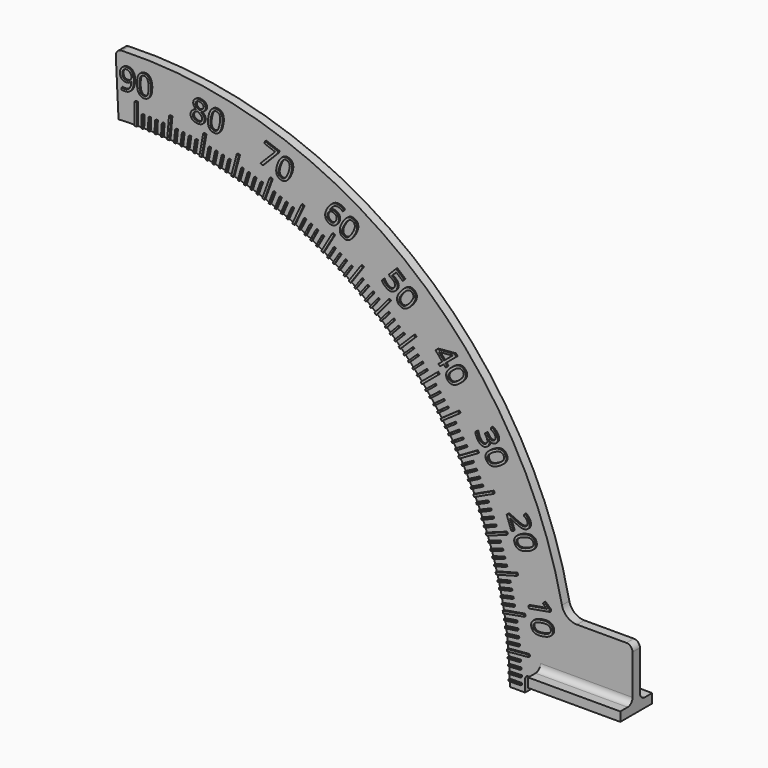
from build123d import *

# Parameters (mm, degrees)
F2_DEPTH     = 1.5
F0_TEXT_SIZE = 9.7222222222
F3_DEPTH     = 2
F4_W         = 30
F4_H         = 3
F5_DEPTH     = 6.5
F6_R         = 2


# Not quite as in the source:
# - Text() gives the source's letters only with a copy of the font that has no kerning and outlines rounded to 1/6400 em; it was checked with that copy


with BuildPart() as f2:
    # F1 (on Front) → F2 (new body, symmetric)
    with BuildSketch(Plane.XZ):
        with BuildLine():
            ThreePointArc((0, 121.5), (85.9134739142, 85.9134739142), (121.5, 0))
            Line((121.5, 0), (126.5, 0))
            Line((126.5, 0), (126.5, 4))
            ThreePointArc((126.5, 4), (126.7928932188, 4.7071067812), (127.5, 5))
            Line((127.5, 5), (161.5, 5))
            Line((161.5, 5), (161.5, 23))
            ThreePointArc((161.5, 23), (160.9142135624, 24.4142135624), (159.5, 25))
            Line((159.5, 25), (143.3954322843, 25))
            ThreePointArc((143.3954322843, 25), (140.2426124294, 26.1193135965), (138.5013902268, 28.976109215))
            ThreePointArc((138.5013902268, 28.976109215), (87.2865254437, 111.3701597196), (-4.9586057544, 141.413090727))
            ThreePointArc((-4.9586057544, 141.413090727), (-6.3611618138, 140.7675835059), (-6.8860808014, 139.315583806))
            Line((-6.8860808014, 139.315583806), (-5.9981707317, 121.3518518519))
            ThreePointArc((-5.9981707317, 121.3518518519), (-3, 121.4629573162), (0, 121.5))
        make_face()
    extrude(amount=F2_DEPTH, both=True)

    # F0 (on Front) → F3 (join)
    with BuildSketch(Plane.XZ):
        with BuildLine():
            ThreePointArc((0.25, 121.4997427981), (0.3000000254, 121.499629629), (0.35, 121.4994958837))
            Line((0.35, 121.4994958837), (0.35, 128.5))
            Line((0.35, 128.5), (-0.35, 128.5))
            Line((-0.35, 128.5), (-0.35, 121.4994958837))
            ThreePointArc((-0.35, 121.4994958837), (-0.3000000254, 121.499629629), (-0.25, 121.4997427981))
            Line((-0.25, 121.4997427981), (-0.25, 125.5))
            Line((-0.25, 125.5), (0.25, 125.5))
            Line((0.25, 125.5), (0.25, 121.4997427981))
        make_face()
        with BuildLine():
            ThreePointArc((1.8705009695, 121.4856009004), (2.1204673821, 121.4814949615), (2.3704248171, 121.4768746971))
            Line((2.3704248171, 121.4768746971), (2.4402389317, 125.4765226405))
            Line((2.4402389317, 125.4765226405), (1.9403150841, 125.4852488437))
            Line((1.9403150841, 125.4852488437), (1.8705009695, 121.4856009004))
        make_face()
        with BuildLine():
            ThreePointArc((3.9904321664, 121.4344533118), (4.2402888494, 121.4259854828), (4.4901275799, 121.4170035634))
            Line((4.4901275799, 121.4170035634), (4.6297345429, 125.4148239167))
            Line((4.6297345429, 125.4148239167), (4.1300391294, 125.4322736651))
            Line((4.1300391294, 125.4322736651), (3.9904321664, 121.4344533118))
        make_face()
        with BuildLine():
            ThreePointArc((6.1091478389, 121.3463156123), (6.3588186835, 121.3334884727), (6.6084626063, 121.3201476342))
            Line((6.6084626063, 121.3201476342), (6.8178198922, 125.3149226226))
            Line((6.8178198922, 125.3149226226), (6.3185051248, 125.3410906008))
            Line((6.3185051248, 125.3410906008), (6.1091478389, 121.3463156123))
        make_face()
        with BuildLine():
            ThreePointArc((8.2260026058, 121.2212146496), (8.4754115599, 121.2040321066), (8.724784631, 121.1863364127))
            Line((8.724784631, 121.1863364127), (9.0038284675, 125.1768491892))
            Line((9.0038284675, 125.1768491892), (8.5050464423, 125.211727426))
            Line((8.5050464423, 125.211727426), (8.2260026058, 121.2212146496))
        make_face()
        with BuildLine():
            ThreePointArc((10.2407106629, 121.0676581302), (10.5894227438, 121.0376558181), (10.9380469515, 121.0066491102))
            Line((10.9380469515, 121.0066491102), (11.5481810874, 127.9805141948))
            Line((11.5481810874, 127.9805141948), (10.8508447987, 128.0415232148))
            Line((10.8508447987, 128.0415232148), (10.2407106629, 121.0676581302))
        make_face()
        with BuildLine():
            ThreePointArc((12.4515509283, 120.8602866101), (12.700208287, 120.8344102872), (12.9488118759, 120.8080223785))
            Line((12.9488118759, 120.8080223785), (13.3669526139, 124.7863657529))
            Line((13.3669526139, 124.7863657529), (12.8696916662, 124.8386299845))
            Line((12.8696916662, 124.8386299845), (12.4515509283, 120.8602866101))
        make_face()
        with BuildLine():
            ThreePointArc((14.5589573408, 120.6245694755), (14.8071252237, 120.5943574244), (15.0552304166, 120.5636348038))
            Line((15.0552304166, 120.5636348038), (15.5427391353, 124.5340746951))
            Line((15.5427391353, 124.5340746951), (15.0464660594, 124.5950093668))
            Line((15.0464660594, 124.5950093668), (14.5589573408, 120.6245694755))
        make_face()
        with BuildLine():
            ThreePointArc((16.6619289539, 120.3521089285), (16.9095317666, 120.3175703521), (17.1570629882, 120.282522378))
            Line((17.1570629882, 120.282522378), (17.7137911877, 124.2438493518))
            Line((17.7137911877, 124.2438493518), (17.2186571533, 124.3134359023))
            Line((17.2186571533, 124.3134359023), (16.6619289539, 120.3521089285))
        make_face()
        with BuildLine():
            ThreePointArc((18.759825182, 120.0429879632), (19.0067875024, 120.0041333823), (19.2536693523, 119.9647707307))
            Line((19.2536693523, 119.9647707307), (19.8794474477, 123.9157781284))
            Line((19.8794474477, 123.9157781284), (19.3856032774, 123.9939953609))
            Line((19.3856032774, 123.9939953609), (18.759825182, 120.0429879632))
        make_face()
        with BuildLine():
            ThreePointArc((20.7534833341, 119.7144223956), (21.0982535865, 119.654141991), (21.4428487612, 119.5928686712))
            Line((21.4428487612, 119.5928686712), (22.6584735438, 126.4870193999))
            Line((22.6584735438, 126.4870193999), (21.9691081166, 126.6085731243))
            Line((21.9691081166, 126.6085731243), (20.7534833341, 119.7144223956))
        make_face()
        with BuildLine():
            ThreePointArc((22.9378370659, 119.3151525613), (23.1832929383, 119.2677027889), (23.4286506577, 119.2197480637))
            Line((23.4286506577, 119.2197480637), (24.1919357156, 123.1465092738))
            Line((24.1919357156, 123.1465092738), (23.7011221239, 123.2419137715))
            Line((23.7011221239, 123.2419137715), (22.9378370659, 119.3151525613))
        make_face()
        with BuildLine():
            ThreePointArc((25.0166800589, 118.8966598304), (25.2612704344, 118.8449334892), (25.5057538593, 118.792703985))
            Line((25.5057538593, 118.792703985), (26.3374540978, 122.7055459694))
            Line((26.3374540978, 122.7055459694), (25.8483802974, 122.8095018148))
            Line((25.8483802974, 122.8095018148), (25.0166800589, 118.8966598304))
        make_face()
        with BuildLine():
            ThreePointArc((27.0879027287, 118.4419500251), (27.3315531028, 118.3859628714), (27.5750877611, 118.329474498))
            Line((27.5750877611, 118.329474498), (28.4749498364, 122.227205367))
            Line((28.4749498364, 122.227205367), (27.987764804, 122.3396808941))
            Line((27.987764804, 122.3396808941), (27.0879027287, 118.4419500251))
        make_face()
        with BuildLine():
            ThreePointArc((29.150874161, 117.9511616545), (29.3935103154, 117.8909307425), (29.6360220242, 117.8302007067))
            Line((29.6360220242, 117.8302007067), (30.6037718293, 121.7116331737))
            Line((30.6037718293, 121.7116331737), (30.1186239662, 121.8325941215))
            Line((30.1186239662, 121.8325941215), (29.150874161, 117.9511616545))
        make_face()
        with BuildLine():
            ThreePointArc((31.1083094659, 117.450087621), (31.44651398, 117.3599878941), (31.7844575443, 117.2689142894))
            Line((31.7844575443, 117.2689142894), (33.5963213349, 124.0308820124))
            Line((33.5963213349, 124.0308820124), (32.9201732565, 124.2120553439))
            Line((32.9201732565, 124.2120553439), (31.1083094659, 117.450087621))
        make_face()
        with BuildLine():
            ThreePointArc((33.2495524133, 116.8619581571), (33.4899387318, 116.7932960565), (33.7301832613, 116.7241394792))
            Line((33.7301832613, 116.7241394792), (34.832803579, 120.5694335013))
            Line((34.832803579, 120.5694335013), (34.352172731, 120.7072521792))
            Line((34.352172731, 120.7072521792), (33.2495524133, 116.8619581571))
        make_face()
        with BuildLine():
            ThreePointArc((35.2840107363, 116.2638748123), (35.5231621238, 116.1910278495), (35.7621631142, 116.1176889599))
            Line((35.7621631142, 116.1176889599), (36.9317251317, 119.9431539472))
            Line((36.9317251317, 119.9431539472), (36.4535727537, 120.0893397995))
            Line((36.4535727537, 120.0893397995), (35.2840107363, 116.2638748123))
        make_face()
        with BuildLine():
            ThreePointArc((37.3077212077, 115.6303763649), (37.5455648166, 115.5533667299), (37.7832494659, 115.4758678677))
            Line((37.7832494659, 115.4758678677), (39.0193969231, 119.2803385464))
            Line((39.0193969231, 119.2803385464), (38.543868665, 119.4348470436))
            Line((38.543868665, 119.4348470436), (37.3077212077, 115.6303763649))
        make_face()
        with BuildLine():
            ThreePointArc((39.3200673859, 114.9616557847), (39.5565307665, 114.8805069353), (39.7928266737, 114.7988717075))
            Line((39.7928266737, 114.7988717075), (41.0951830283, 118.5811891991))
            Line((41.0951830283, 118.5811891991), (40.6224237405, 118.7439732763))
            Line((40.6224237405, 118.7439732763), (39.3200673859, 114.9616557847))
        make_face()
        with BuildLine():
            ThreePointArc((41.2263825789, 114.2918867613), (41.5554474141, 114.1726534255), (41.8841674134, 114.052472661))
            Line((41.8841674134, 114.052472661), (44.2784808346, 120.6307947208))
            Line((44.2784808346, 120.6307947208), (43.620696, 120.8702088212))
            Line((43.620696, 120.8702088212), (41.2263825789, 114.2918867613))
        make_face()
        with BuildLine():
            ThreePointArc((43.3082185902, 113.5193736881), (43.5417058698, 113.4300218194), (43.7750088035, 113.3401897133))
            Line((43.7750088035, 113.3401897133), (45.2085727746, 117.074751538))
            Line((45.2085727746, 117.074751538), (44.7417825613, 117.2539355128))
            Line((44.7417825613, 117.2539355128), (43.3082185902, 113.5193736881))
        make_face()
        with BuildLine():
            ThreePointArc((45.2828087869, 112.7462515048), (45.5147011, 112.6528383299), (45.7464007141, 112.558948208))
            Line((45.7464007141, 112.558948208), (47.2449234373, 116.2679220998))
            Line((47.2449234373, 116.2679220998), (46.7813315101, 116.4552253965))
            Line((46.7813315101, 116.4552253965), (45.2828087869, 112.7462515048))
        make_face()
        with BuildLine():
            ThreePointArc((47.2436054013, 111.938785721), (47.4738321114, 111.8413396945), (47.703857828, 111.7434201567))
            Line((47.703857828, 111.7434201567), (49.2668828388, 115.4256763262))
            Line((49.2668828388, 115.4256763262), (48.806630412, 115.6210418904))
            Line((48.806630412, 115.6210418904), (47.2436054013, 111.938785721))
        make_face()
        with BuildLine():
            ThreePointArc((49.1900111559, 111.0972222987), (49.4185021337, 110.9957731036), (49.6467838847, 110.8938539772))
            Line((49.6467838847, 110.8938539772), (51.2738350704, 114.5482707734))
            Line((51.2738350704, 114.5482707734), (50.8170623416, 114.7516390949))
            Line((50.8170623416, 114.7516390949), (49.1900111559, 111.0972222987))
        make_face()
        with BuildLine():
            ThreePointArc((51.0306980273, 110.2638556321), (51.3481188015, 110.116396125), (51.6651134782, 109.9680228488))
            Line((51.6651134782, 109.9680228488), (54.6236543591, 116.3126342426))
            Line((54.6236543591, 116.3126342426), (53.9892389082, 116.6084670258))
            Line((53.9892389082, 116.6084670258), (51.0306980273, 110.2638556321))
        make_face()
        with BuildLine():
            ThreePointArc((53.0372830734, 109.3128382405), (53.2620943349, 109.2034766253), (53.4866800965, 109.0936526671))
            Line((53.4866800965, 109.0936526671), (55.2402774336, 112.6890600238))
            Line((55.2402774336, 112.6890600238), (54.7908804105, 112.9082455972))
            Line((54.7908804105, 112.9082455972), (53.0372830734, 109.3128382405))
        make_face()
        with BuildLine():
            ThreePointArc((54.9369773201, 108.3705611452), (55.1598457184, 108.2572926889), (55.3824805822, 108.1435658954))
            Line((55.3824805822, 108.1435658954), (57.1985593484, 111.7078211607))
            Line((57.1985593484, 111.7078211607), (56.7530560863, 111.9348164106))
            Line((56.7530560863, 111.9348164106), (54.9369773201, 108.3705611452))
        make_face()
        with BuildLine():
            ThreePointArc((56.8199372313, 107.3952733272), (57.0407948785, 107.2781325324), (57.2614110277, 107.1605375458))
            Line((57.2614110277, 107.1605375458), (59.1394180278, 110.6925550131))
            Line((59.1394180278, 110.6925550131), (58.6979442314, 110.9272907945))
            Line((58.6979442314, 110.9272907945), (56.8199372313, 107.3952733272))
        make_face()
        with BuildLine():
            ThreePointArc((58.6855892392, 106.3872718686), (58.9043688599, 106.2662944174), (59.1228990928, 106.1448670585))
            Line((59.1228990928, 106.1448670585), (61.0622622677, 109.6435708409))
            Line((61.0622622677, 109.6435708409), (60.6249524141, 109.8859756511))
            Line((60.6249524141, 109.8859756511), (58.6855892392, 106.3872718686))
        make_face()
        with BuildLine():
            ThreePointArc((60.4466390505, 105.3966499823), (60.75, 105.2220865598), (61.0528568332, 105.0466499823))
            Line((61.0528568332, 105.0466499823), (64.5531088913, 111.1092643863))
            Line((64.5531088913, 111.1092643863), (63.9468911087, 111.4592643863))
            Line((63.9468911087, 111.4592643863), (60.4466390505, 105.3966499823))
        make_face()
        with BuildLine():
            ThreePointArc((62.3627018076, 104.274366089), (62.5771261016, 104.1458270353), (62.791285458, 104.0168470515))
            Line((62.791285458, 104.0168470515), (64.8515702264, 107.4457367194))
            Line((64.8515702264, 107.4457367194), (64.422986576, 107.7032557568))
            Line((64.422986576, 107.7032557568), (62.3627018076, 104.274366089))
        make_face()
        with BuildLine():
            ThreePointArc((64.173042284, 103.1701053795), (64.3851906043, 103.037843683), (64.5970663321, 102.9051457474))
            Line((64.5970663321, 102.9051457474), (66.7168796853, 106.2975562516))
            Line((66.7168796853, 106.2975562516), (66.2928556372, 106.5625158837))
            Line((66.2928556372, 106.5625158837), (64.173042284, 103.1701053795))
        make_face()
        with BuildLine():
            ThreePointArc((65.9638350301, 102.0344180564), (66.1736427543, 101.8984740054), (66.3831703141, 101.7620985389))
            Line((66.3831703141, 101.7620985389), (68.5618665364, 105.1169965184))
            Line((68.5618665364, 105.1169965184), (68.1425312524, 105.3893160359))
            Line((68.1425312524, 105.3893160359), (65.9638350301, 102.0344180564))
        make_face()
        with BuildLine():
            ThreePointArc((67.7345345531, 100.8676500613), (67.9419377717, 100.7280650654), (68.1490533393, 100.5880536095))
            Line((68.1490533393, 100.5880536095), (70.3859687787, 103.9044171298))
            Line((70.3859687787, 103.9044171298), (69.9714499924, 104.1840135815))
            Line((69.9714499924, 104.1840135815), (67.7345345531, 100.8676500613))
        make_face()
        with BuildLine():
            ThreePointArc((69.4025446519, 99.727312186), (69.6895370167, 99.5269733811), (69.9759510829, 99.3258086805))
            Line((69.9759510829, 99.3258086805), (73.9912752866, 105.0602859384))
            Line((73.9912752866, 105.0602859384), (73.4178688556, 105.4617894439))
            Line((73.4178688556, 105.4617894439), (69.4025446519, 99.727312186))
        make_face()
        with BuildLine():
            ThreePointArc((71.2135027254, 98.4423030489), (71.4159081535, 98.2955648166), (71.6180112226, 98.1484104228))
            Line((71.6180112226, 98.1484104228), (73.9693034113, 101.384686481))
            Line((73.9693034113, 101.384686481), (73.5647949141, 101.6785791071))
            Line((73.5647949141, 101.6785791071), (71.2135027254, 98.4423030489))
        make_face()
        with BuildLine():
            ThreePointArc((72.9207116475, 97.1844628159), (73.120525313, 97.0342144707), (73.3200294025, 96.8835553044))
            Line((73.3200294025, 96.8835553044), (75.7274442831, 100.0783027551))
            Line((75.7274442831, 100.0783027551), (75.3281265281, 100.3792102667))
            Line((75.3281265281, 100.3792102667), (72.9207116475, 97.1844628159))
        make_face()
        with BuildLine():
            ThreePointArc((74.6057082144, 95.8970192542), (74.8028692521, 95.7433065632), (74.9997135912, 95.5891885165))
            Line((74.9997135912, 95.5891885165), (77.4625178418, 98.7414342088))
            Line((77.4625178418, 98.7414342088), (77.068512465, 99.0492649465))
            Line((77.068512465, 99.0492649465), (74.6057082144, 95.8970192542))
        make_face()
        with BuildLine():
            ThreePointArc((76.2679791598, 94.5803645314), (76.4624275126, 94.423234317), (76.6565521405, 94.2657043358))
            Line((76.6565521405, 94.2657043358), (79.1739955671, 97.3744880651))
            Line((79.1739955671, 97.3744880651), (78.7854225864, 97.6891482606))
            Line((78.7854225864, 97.6891482606), (76.2679791598, 94.5803645314))
        make_face()
        with BuildLine():
            ThreePointArc((77.8302549821, 93.2989893269), (78.0986945769, 93.0743998389), (78.3664860924, 92.8490380001))
            Line((78.3664860923, 92.849038), (82.8663233998, 98.2117352774))
            Line((82.8663233998, 98.2117352774), (82.3300922896, 98.6616866042))
            Line((82.3300922896, 98.6616866042), (77.8302549821, 93.2989893269))
        make_face()
        with BuildLine():
            ThreePointArc((79.5223258877, 91.8610346416), (79.7111720223, 91.6972139971), (79.8996806778, 91.5330051271))
            Line((79.8996806778, 91.5330051271), (82.5240855334, 94.5520375607))
            Line((82.5240855334, 94.5520375607), (82.1467307433, 94.8800670752))
            Line((82.1467307433, 94.8800670752), (79.5223258877, 91.8610346416))
        make_face()
        with BuildLine():
            ThreePointArc((81.1134103646, 90.4591878088), (81.2993686726, 90.2920962955), (81.4849827773, 90.1246225056))
            Line((81.4849827773, 90.1246225056), (84.1616773044, 93.0973929458))
            Line((84.1616773044, 93.0973929458), (83.7901048917, 93.431958249))
            Line((83.7901048917, 93.431958249), (81.1134103646, 90.4591878088))
        make_face()
        with BuildLine():
            ThreePointArc((82.6797869109, 89.0297862312), (82.8628007476, 88.8594747467), (83.0454637617, 88.6887870511))
            Line((83.0454637617, 88.6887870511), (85.7736326132, 91.6143899632))
            Line((85.7736326132, 91.6143899632), (85.4079557624, 91.9553891432))
            Line((85.4079557624, 91.9553891432), (82.6797869109, 89.0297862312))
        make_face()
        with BuildLine():
            ThreePointArc((84.2209783932, 87.5732653182), (84.4009920108, 87.3997857411), (84.5806482934, 87.225936133))
            Line((84.5806482934, 87.225936133), (87.3594604427, 90.1034803499))
            Line((87.3594604427, 90.1034803499), (86.9997905425, 90.4508095351))
            Line((86.9997905425, 90.4508095351), (84.2209783932, 87.5732653182))
        make_face()
        with BuildLine():
            ThreePointArc((85.6656300767, 86.1606048235), (85.9134739142, 85.9134739142), (86.1606048235, 85.6656300767))
            Line((86.1606048235, 85.6656300767), (91.1107087559, 90.6157340091))
            Line((91.1107087559, 90.6157340091), (90.6157340091, 91.1107087559))
            Line((90.6157340091, 91.1107087559), (85.6656300767, 86.1606048235))
        make_face()
        with BuildLine():
            ThreePointArc((87.225936133, 84.5806482934), (87.3997857411, 84.4009920108), (87.5732653182, 84.2209783932))
            Line((87.5732653182, 84.2209783932), (90.4508095351, 86.9997905425))
            Line((90.4508095351, 86.9997905425), (90.1034803499, 87.3594604427))
            Line((90.1034803499, 87.3594604427), (87.225936133, 84.5806482934))
        make_face()
        with BuildLine():
            ThreePointArc((88.6887870511, 83.0454637617), (88.8594747467, 82.8628007476), (89.0297862312, 82.6797869109))
            Line((89.0297862312, 82.6797869109), (91.9553891432, 85.4079557624))
            Line((91.9553891432, 85.4079557624), (91.6143899632, 85.7736326132))
            Line((91.6143899632, 85.7736326132), (88.6887870511, 83.0454637617))
        make_face()
        with BuildLine():
            ThreePointArc((90.1246225056, 81.4849827773), (90.2920962955, 81.2993686726), (90.4591878088, 81.1134103646))
            Line((90.4591878088, 81.1134103646), (93.431958249, 83.7901048917))
            Line((93.431958249, 83.7901048917), (93.0973929458, 84.1616773044))
            Line((93.0973929458, 84.1616773044), (90.1246225056, 81.4849827773))
        make_face()
        with BuildLine():
            ThreePointArc((91.5330051271, 79.8996806778), (91.6972139971, 79.7111720223), (91.8610346416, 79.5223258877))
            Line((91.8610346416, 79.5223258877), (94.8800670752, 82.1467307433))
            Line((94.8800670752, 82.1467307433), (94.5520375607, 82.5240855334))
            Line((94.5520375607, 82.5240855334), (91.5330051271, 79.8996806778))
        make_face()
        with BuildLine():
            ThreePointArc((92.8490380001, 78.3664860924), (93.0743998389, 78.0986945769), (93.2989893269, 77.8302549821))
            Line((93.2989893269, 77.8302549821), (98.6616866042, 82.3300922896))
            Line((98.6616866042, 82.3300922896), (98.2117352774, 82.8663233998))
            Line((98.2117352774, 82.8663233998), (92.849038, 78.3664860923))
        make_face()
        with BuildLine():
            ThreePointArc((94.2657043358, 76.6565521405), (94.423234317, 76.4624275126), (94.5803645314, 76.2679791598))
            Line((94.5803645314, 76.2679791598), (97.6891482606, 78.7854225864))
            Line((97.6891482606, 78.7854225864), (97.3744880651, 79.1739955671))
            Line((97.3744880651, 79.1739955671), (94.2657043358, 76.6565521405))
        make_face()
        with BuildLine():
            ThreePointArc((95.5891885165, 74.9997135912), (95.7433065632, 74.8028692521), (95.8970192542, 74.6057082144))
            Line((95.8970192542, 74.6057082144), (99.0492649465, 77.068512465))
            Line((99.0492649465, 77.068512465), (98.7414342088, 77.4625178418))
            Line((98.7414342088, 77.4625178418), (95.5891885165, 74.9997135912))
        make_face()
        with BuildLine():
            ThreePointArc((96.8835553044, 73.3200294025), (97.0342144707, 73.120525313), (97.1844628159, 72.9207116475))
            Line((97.1844628159, 72.9207116475), (100.3792102667, 75.3281265281))
            Line((100.3792102667, 75.3281265281), (100.0783027551, 75.7274442831))
            Line((100.0783027551, 75.7274442831), (96.8835553044, 73.3200294025))
        make_face()
        with BuildLine():
            ThreePointArc((98.1484104228, 71.6180112226), (98.2955648166, 71.4159081535), (98.4423030489, 71.2135027254))
            Line((98.4423030489, 71.2135027254), (101.6785791071, 73.5647949141))
            Line((101.6785791071, 73.5647949141), (101.384686481, 73.9693034113))
            Line((101.384686481, 73.9693034113), (98.1484104228, 71.6180112226))
        make_face()
        with BuildLine():
            ThreePointArc((99.3258086805, 69.9759510829), (99.5269733811, 69.6895370167), (99.727312186, 69.4025446519))
            Line((99.727312186, 69.4025446519), (105.4617894439, 73.4178688556))
            Line((105.4617894439, 73.4178688556), (105.0602859384, 73.9912752866))
            Line((105.0602859384, 73.9912752866), (99.3258086805, 69.9759510829))
        make_face()
        with BuildLine():
            ThreePointArc((100.5880536095, 68.1490533393), (100.7280650654, 67.9419377717), (100.8676500613, 67.7345345531))
            Line((100.8676500613, 67.7345345531), (104.1840135815, 69.9714499924))
            Line((104.1840135815, 69.9714499924), (103.9044171298, 70.3859687787))
            Line((103.9044171298, 70.3859687787), (100.5880536095, 68.1490533393))
        make_face()
        with BuildLine():
            ThreePointArc((101.7620985389, 66.3831703141), (101.8984740054, 66.1736427543), (102.0344180564, 65.9638350301))
            Line((102.0344180564, 65.9638350301), (105.3893160359, 68.1425312524))
            Line((105.3893160359, 68.1425312524), (105.1169965184, 68.5618665364))
            Line((105.1169965184, 68.5618665364), (101.7620985389, 66.3831703141))
        make_face()
        with BuildLine():
            ThreePointArc((102.9051457474, 64.5970663321), (103.037843683, 64.3851906043), (103.1701053795, 64.173042284))
            Line((103.1701053795, 64.173042284), (106.5625158837, 66.2928556372))
            Line((106.5625158837, 66.2928556372), (106.2975562516, 66.7168796853))
            Line((106.2975562516, 66.7168796853), (102.9051457474, 64.5970663321))
        make_face()
        with BuildLine():
            ThreePointArc((104.0168470515, 62.791285458), (104.1458270353, 62.5771261016), (104.274366089, 62.3627018076))
            Line((104.274366089, 62.3627018076), (107.7032557568, 64.422986576))
            Line((107.7032557568, 64.422986576), (107.4457367194, 64.8515702264))
            Line((107.4457367194, 64.8515702264), (104.0168470515, 62.791285458))
        make_face()
        with BuildLine():
            ThreePointArc((105.0466499823, 61.0528568332), (105.2220865598, 60.75), (105.3966499823, 60.4466390505))
            Line((105.3966499823, 60.4466390505), (111.4592643863, 63.9468911087))
            Line((111.4592643863, 63.9468911087), (111.1092643863, 64.5531088913))
            Line((111.1092643863, 64.5531088913), (105.0466499823, 61.0528568332))
        make_face()
        with BuildLine():
            ThreePointArc((106.1448670585, 59.1228990928), (106.2662944174, 58.9043688599), (106.3872718686, 58.6855892392))
            Line((106.3872718686, 58.6855892392), (109.8859756511, 60.6249524141))
            Line((109.8859756511, 60.6249524141), (109.6435708409, 61.0622622677))
            Line((109.6435708409, 61.0622622677), (106.1448670585, 59.1228990928))
        make_face()
        with BuildLine():
            ThreePointArc((107.1605375458, 57.2614110277), (107.2781325324, 57.0407948785), (107.3952733272, 56.8199372313))
            Line((107.3952733272, 56.8199372313), (110.9272907945, 58.6979442314))
            Line((110.9272907945, 58.6979442314), (110.6925550131, 59.1394180278))
            Line((110.6925550131, 59.1394180278), (107.1605375458, 57.2614110277))
        make_face()
        with BuildLine():
            ThreePointArc((108.1435658954, 55.3824805822), (108.2572926889, 55.1598457184), (108.3705611452, 54.9369773201))
            Line((108.3705611452, 54.9369773201), (111.9348164106, 56.7530560863))
            Line((111.9348164106, 56.7530560863), (111.7078211607, 57.1985593484))
            Line((111.7078211607, 57.1985593484), (108.1435658954, 55.3824805822))
        make_face()
        with BuildLine():
            ThreePointArc((109.0936526671, 53.4866800965), (109.2034766253, 53.2620943349), (109.3128382405, 53.0372830734))
            Line((109.3128382405, 53.0372830734), (112.9082455972, 54.7908804105))
            Line((112.9082455972, 54.7908804105), (112.6890600238, 55.2402774336))
            Line((112.6890600238, 55.2402774336), (109.0936526671, 53.4866800965))
        make_face()
        with BuildLine():
            ThreePointArc((109.9680228488, 51.6651134782), (110.116396125, 51.3481188015), (110.2638556321, 51.0306980273))
            Line((110.2638556321, 51.0306980273), (116.6084670258, 53.9892389082))
            Line((116.6084670258, 53.9892389082), (116.3126342426, 54.6236543591))
            Line((116.3126342426, 54.6236543591), (109.9680228488, 51.6651134782))
        make_face()
        with BuildLine():
            ThreePointArc((110.8938539772, 49.6467838847), (110.9957731036, 49.4185021337), (111.0972222987, 49.1900111559))
            Line((111.0972222987, 49.1900111559), (114.7516390949, 50.8170623416))
            Line((114.7516390949, 50.8170623416), (114.5482707734, 51.2738350704))
            Line((114.5482707734, 51.2738350704), (110.8938539772, 49.6467838847))
        make_face()
        with BuildLine():
            ThreePointArc((111.7434201567, 47.703857828), (111.8413396945, 47.4738321114), (111.938785721, 47.2436054013))
            Line((111.938785721, 47.2436054013), (115.6210418904, 48.806630412))
            Line((115.6210418904, 48.806630412), (115.4256763262, 49.2668828388))
            Line((115.4256763262, 49.2668828388), (111.7434201567, 47.703857828))
        make_face()
        with BuildLine():
            ThreePointArc((112.558948208, 45.7464007141), (112.6528383299, 45.5147011), (112.7462515048, 45.2828087869))
            Line((112.7462515048, 45.2828087869), (116.4552253965, 46.7813315101))
            Line((116.4552253965, 46.7813315101), (116.2679220998, 47.2449234373))
            Line((116.2679220998, 47.2449234373), (112.558948208, 45.7464007141))
        make_face()
        with BuildLine():
            ThreePointArc((113.3401897133, 43.7750088035), (113.4300218194, 43.5417058698), (113.5193736881, 43.3082185902))
            Line((113.5193736881, 43.3082185902), (117.2539355128, 44.7417825613))
            Line((117.2539355128, 44.7417825613), (117.074751538, 45.2085727746))
            Line((117.074751538, 45.2085727746), (113.3401897133, 43.7750088035))
        make_face()
        with BuildLine():
            ThreePointArc((114.052472661, 41.8841674134), (114.1726534255, 41.5554474141), (114.2918867613, 41.2263825789))
            Line((114.2918867613, 41.2263825789), (120.8702088212, 43.620696))
            Line((120.8702088212, 43.620696), (120.6307947208, 44.2784808346))
            Line((120.6307947208, 44.2784808346), (114.052472661, 41.8841674134))
        make_face()
        with BuildLine():
            ThreePointArc((114.7988717075, 39.7928266737), (114.8805069353, 39.5565307665), (114.9616557847, 39.3200673859))
            Line((114.9616557847, 39.3200673859), (118.7439732763, 40.6224237405))
            Line((118.7439732763, 40.6224237405), (118.5811891991, 41.0951830283))
            Line((118.5811891991, 41.0951830283), (114.7988717075, 39.7928266737))
        make_face()
        with BuildLine():
            ThreePointArc((115.4758678677, 37.7832494659), (115.5533667299, 37.5455648166), (115.6303763649, 37.3077212077))
            Line((115.6303763649, 37.3077212077), (119.4348470436, 38.543868665))
            Line((119.4348470436, 38.543868665), (119.2803385464, 39.0193969231))
            Line((119.2803385464, 39.0193969231), (115.4758678677, 37.7832494659))
        make_face()
        with BuildLine():
            ThreePointArc((116.1176889599, 35.7621631142), (116.1910278495, 35.5231621238), (116.2638748123, 35.2840107363))
            Line((116.2638748123, 35.2840107363), (120.0893397995, 36.4535727537))
            Line((120.0893397995, 36.4535727537), (119.9431539472, 36.9317251317))
            Line((119.9431539472, 36.9317251317), (116.1176889599, 35.7621631142))
        make_face()
        with BuildLine():
            ThreePointArc((116.7241394792, 33.7301832613), (116.7932960565, 33.4899387318), (116.8619581571, 33.2495524133))
            Line((116.8619581571, 33.2495524133), (120.7072521792, 34.352172731))
            Line((120.7072521792, 34.352172731), (120.5694335013, 34.832803579))
            Line((120.5694335013, 34.832803579), (116.7241394792, 33.7301832613))
        make_face()
        with BuildLine():
            ThreePointArc((117.2689142894, 31.7844575443), (117.3599878941, 31.44651398), (117.450087621, 31.1083094659))
            Line((117.450087621, 31.1083094659), (124.2120553439, 32.9201732565))
            Line((124.2120553439, 32.9201732565), (124.0308820124, 33.5963213349))
            Line((124.0308820124, 33.5963213349), (117.2689142894, 31.7844575443))
        make_face()
        with BuildLine():
            ThreePointArc((117.8302007067, 29.6360220242), (117.8909307425, 29.3935103154), (117.9511616545, 29.150874161))
            Line((117.9511616545, 29.150874161), (121.8325941215, 30.1186239662))
            Line((121.8325941215, 30.1186239662), (121.7116331737, 30.6037718293))
            Line((121.7116331737, 30.6037718293), (117.8302007067, 29.6360220242))
        make_face()
        with BuildLine():
            ThreePointArc((118.329474498, 27.5750877611), (118.3859628714, 27.3315531028), (118.4419500251, 27.0879027287))
            Line((118.4419500251, 27.0879027287), (122.3396808941, 27.987764804))
            Line((122.3396808941, 27.987764804), (122.227205367, 28.4749498364))
            Line((122.227205367, 28.4749498364), (118.329474498, 27.5750877611))
        make_face()
        with BuildLine():
            ThreePointArc((118.792703985, 25.5057538593), (118.8449334892, 25.2612704344), (118.8966598304, 25.0166800589))
            Line((118.8966598304, 25.0166800589), (122.8095018148, 25.8483802974))
            Line((122.8095018148, 25.8483802974), (122.7055459694, 26.3374540978))
            Line((122.7055459694, 26.3374540978), (118.792703985, 25.5057538593))
        make_face()
        with BuildLine():
            ThreePointArc((119.2197480637, 23.4286506577), (119.2677027889, 23.1832929383), (119.3151525613, 22.9378370659))
            Line((119.3151525613, 22.9378370659), (123.2419137715, 23.7011221239))
            Line((123.2419137715, 23.7011221239), (123.1465092738, 24.1919357156))
            Line((123.1465092738, 24.1919357156), (119.2197480637, 23.4286506577))
        make_face()
        with BuildLine():
            ThreePointArc((119.5928686712, 21.4428487612), (119.654141991, 21.0982535865), (119.7144223956, 20.7534833341))
            Line((119.7144223956, 20.7534833341), (126.6085731243, 21.9691081166))
            Line((126.6085731243, 21.9691081166), (126.4870193999, 22.6584735438))
            Line((126.4870193999, 22.6584735438), (119.5928686712, 21.4428487612))
        make_face()
        with BuildLine():
            ThreePointArc((119.9647707307, 19.2536693523), (120.0041333823, 19.0067875024), (120.0429879632, 18.759825182))
            Line((120.0429879632, 18.759825182), (123.9939953609, 19.3856032774))
            Line((123.9939953609, 19.3856032774), (123.9157781284, 19.8794474477))
            Line((123.9157781284, 19.8794474477), (119.9647707307, 19.2536693523))
        make_face()
        with BuildLine():
            ThreePointArc((120.282522378, 17.1570629882), (120.3175703521, 16.9095317666), (120.3521089285, 16.6619289539))
            Line((120.3521089285, 16.6619289539), (124.3134359023, 17.2186571533))
            Line((124.3134359023, 17.2186571533), (124.2438493518, 17.7137911877))
            Line((124.2438493518, 17.7137911877), (120.282522378, 17.1570629882))
        make_face()
        with BuildLine():
            ThreePointArc((120.5636348038, 15.0552304166), (120.5943574244, 14.8071252237), (120.6245694755, 14.5589573408))
            Line((120.6245694755, 14.5589573408), (124.5950093668, 15.0464660594))
            Line((124.5950093668, 15.0464660594), (124.5340746951, 15.5427391353))
            Line((124.5340746951, 15.5427391353), (120.5636348038, 15.0552304166))
        make_face()
        with BuildLine():
            ThreePointArc((120.8080223785, 12.9488118759), (120.8344102872, 12.700208287), (120.8602866101, 12.4515509283))
            Line((120.8602866101, 12.4515509283), (124.8386299845, 12.8696916662))
            Line((124.8386299845, 12.8696916662), (124.7863657529, 13.3669526139))
            Line((124.7863657529, 13.3669526139), (120.8080223785, 12.9488118759))
        make_face()
        with BuildLine():
            ThreePointArc((121.0066491102, 10.9380469515), (121.0376558181, 10.5894227438), (121.0676581302, 10.2407106629))
            Line((121.0676581302, 10.2407106629), (128.0415232148, 10.8508447987))
            Line((128.0415232148, 10.8508447987), (127.9805141948, 11.5481810874))
            Line((127.9805141948, 11.5481810874), (121.0066491102, 10.9380469515))
        make_face()
        with BuildLine():
            ThreePointArc((121.1863364127, 8.724784631), (121.2040321066, 8.4754115599), (121.2212146496, 8.2260026058))
            Line((121.2212146496, 8.2260026058), (125.211727426, 8.5050464423))
            Line((125.211727426, 8.5050464423), (125.1768491892, 9.0038284675))
            Line((125.1768491892, 9.0038284675), (121.1863364127, 8.724784631))
        make_face()
        with BuildLine():
            ThreePointArc((121.3201476342, 6.6084626063), (121.3334884727, 6.3588186835), (121.3463156123, 6.1091478389))
            Line((121.3463156123, 6.1091478389), (125.3410906008, 6.3185051248))
            Line((125.3410906008, 6.3185051248), (125.3149226226, 6.8178198922))
            Line((125.3149226226, 6.8178198922), (121.3201476342, 6.6084626063))
        make_face()
        with BuildLine():
            ThreePointArc((121.4170035634, 4.4901275799), (121.4259854828, 4.2402888494), (121.4344533118, 3.9904321664))
            Line((121.4344533118, 3.9904321664), (125.4322736651, 4.1300391294))
            Line((125.4322736651, 4.1300391294), (125.4148239167, 4.6297345429))
            Line((125.4148239167, 4.6297345429), (121.4170035634, 4.4901275799))
        make_face()
        with BuildLine():
            ThreePointArc((121.4768746971, 2.3704248171), (121.4814949615, 2.1204673821), (121.4856009004, 1.8705009695))
            Line((121.4856009004, 1.8705009695), (125.4852488437, 1.9403150841))
            Line((125.4852488437, 1.9403150841), (125.4765226405, 2.4402389317))
            Line((125.4765226405, 2.4402389317), (121.4768746971, 2.3704248171))
        make_face()
        with BuildLine():
            ThreePointArc((0, 121.5), (0.1250000662, 121.4999356995), (0.25, 121.4997427981))
            Line((0.25, 121.4997427981), (0.25, 125.5))
            Line((0.25, 125.5), (-0.25, 125.5))
            Line((-0.25, 125.5), (-0.25, 121.4997427981))
            ThreePointArc((-0.25, 121.4997427981), (-0.1250000662, 121.4999356995), (0, 121.5))
        make_face()
        with Locations((-5.6320529514, 130.5)):
            Text('90', F0_TEXT_SIZE, font='Open Sans', text_align=(TextAlign.LEFT, TextAlign.BOTTOM))
        with Locations(Location((17.1145977736, 129.4954074996), (0, 0, -10))):
            Text('80', F0_TEXT_SIZE, font='Open Sans', text_align=(TextAlign.LEFT, TextAlign.BOTTOM))
        with Locations(Location((39.3412301057, 124.5561625702), (0, 0, -20))):
            Text('70', F0_TEXT_SIZE, font='Open Sans', text_align=(TextAlign.LEFT, TextAlign.BOTTOM))
        with Locations(Location((60.3724990686, 115.8323416696), (0, 0, -30))):
            Text('60', F0_TEXT_SIZE, font='Open Sans', text_align=(TextAlign.LEFT, TextAlign.BOTTOM))
        with Locations(Location((79.5693801973, 103.5890136813), (0, 0, -40))):
            Text('50', F0_TEXT_SIZE, font='Open Sans', text_align=(TextAlign.LEFT, TextAlign.BOTTOM))
        with Locations(Location((96.3485859728, 88.1981859309), (0, 0, -50))):
            Text('40', F0_TEXT_SIZE, font='Open Sans', text_align=(TextAlign.LEFT, TextAlign.BOTTOM))
        with Locations(Location((110.2002887182, 70.1275009314), (0, 0, -60))):
            Text('30', F0_TEXT_SIZE, font='Open Sans', text_align=(TextAlign.LEFT, TextAlign.BOTTOM))
        with Locations(Location((120.7036114549, 49.9260273023), (0, 0, -70))):
            Text('20', F0_TEXT_SIZE, font='Open Sans', text_align=(TextAlign.LEFT, TextAlign.BOTTOM))
        with Locations(Location((127.5394160366, 28.2075765974), (0, 0, -80))):
            Text('10', F0_TEXT_SIZE, font='Open Sans', text_align=(TextAlign.LEFT, TextAlign.BOTTOM))
    extrude(amount=F3_DEPTH)

    # F4 (on Front) → F5 (join, symmetric)
    with BuildSketch(Plane.XZ):
        with Locations((146.5, 6.5)):
            Rectangle(F4_W, F4_H)
    extrude(amount=F5_DEPTH, both=True)

    # F6
    f6_edges = [f2.edges().sort_by_distance(p)[0] for p in [
        (146.5, 1.5, 8),
        (146.5, -1.5, 8),
    ]]
    fillet(f6_edges, radius=F6_R)


solid = f2.part
